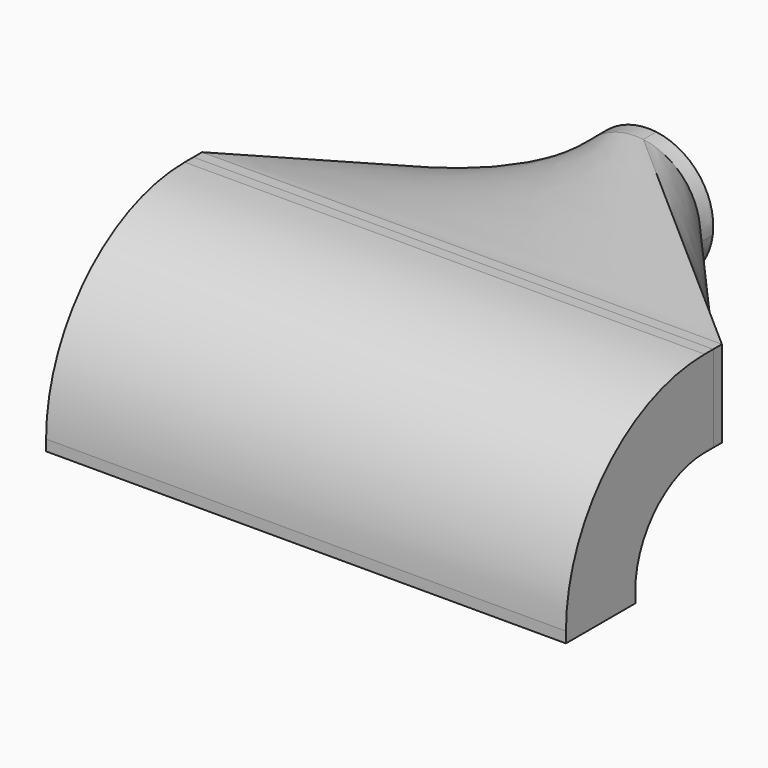
from build123d import *

# Parameters (mm, degrees)
F0_W      = 1828.8
F0_H      = 304.8
F1_DEPTH  = 38.1
F2_W      = 1828.8
F2_H      = 304.8
F3_ANGLE  = 90
F4_DEPTH  = 38.1
F5_W      = 1828.8
F5_H      = 304.8
F6_DEPTH  = 38.1
F6_FACE_W = 1828.8
F6_FACE_H = 304.8
F10_DEPTH = 57.15


# Not quite as in the source:
# - the arcs of a loft's sections are written as splines that run evenly, so that the points pair up as in the source's solid


with BuildPart() as f1:
    # F0 (on Top) → F1 (new body)
    with BuildSketch(Plane.XY):
        Rectangle(F0_W, F0_H)
    extrude(amount=F1_DEPTH)

    # F2 (on face) → F3 (revolve)
    with BuildSketch(Plane.XY.offset(38.1)):
        Rectangle(F2_W, F2_H)
    revolve(axis=Axis((-103.2055318356, 457.2, 38.1), (-1, 0, 0)), revolution_arc=F3_ANGLE)

    # F4 (add): a face of the model
    f4_faces = [f1.faces().sort_by_distance(p)[0] for p in [
        (0, 457.2, 495.3),
    ]]
    extrude(f4_faces, amount=F4_DEPTH)


with BuildPart() as f6:
    # F5 (on face) → F6 (new body)
    with BuildSketch(Plane(origin=(0, 495.3, 0), x_dir=(-1, 0, 0), z_dir=(0, 1, 0))):
        with Locations((0, 495.3)):
            Rectangle(F5_W, F5_H)
    extrude(amount=F6_DEPTH)

    # F6_face (on face) → F9 section 0
    with BuildSketch(Plane(origin=(0, 533.4, 495.3), x_dir=(-1, 0, 0), z_dir=(0, 1, 0))):
        Rectangle(F6_FACE_W, F6_FACE_H)
    # F8 (on offset) → F9 section 1
    with BuildSketch(Plane(origin=(0, 1295.4, 0), x_dir=(-1, 0, 0), z_dir=(0, 1, 0))):
        with BuildLine():
            add(Edge.make_bspline(
                [(-226.8347226167, 428.8456596729), (-224.978935382, 413.9993617947), (-221.6609974791, 399.3362055901), (-212.2280018047, 370.9382369937), (-206.1131772825, 357.2041267978), (-191.3212651368, 331.1921033689), (-182.6445432725, 318.9148333344), (-163.062159544, 296.2883825456), (-152.1569818928, 285.9397612748), (-128.5366666062, 267.5684049408), (-115.8221130296, 259.5461241455), (-89.0715816549, 246.1358631874), (-75.0362653164, 240.7482146197), (-46.1835257726, 232.8143978457), (-31.366816008, 230.2684258186), (-1.5206628948, 228.1159453578), (13.5080424489, 228.5094901485), (28.3543403271, 230.3652773833)],
                knots=[0, 0, 0, 0, 0.125, 0.125, 0.25, 0.25, 0.375, 0.375, 0.5, 0.5, 0.625, 0.625, 0.75, 0.75, 0.875, 0.875, 1, 1, 1, 1], degree=3))
            add(Edge.make_bspline(
                [(28.3543403271, 230.3652773833), (43.2006382053, 232.221064618), (57.8637944099, 235.5390025209), (86.2617630063, 244.9719981953), (99.9958732022, 251.0868227175), (126.0078966311, 265.8787348632), (138.2851666656, 274.5554567275), (160.9116174544, 294.137840456), (171.2602387252, 305.0430181072), (189.6315950592, 328.6633333938), (197.6538758545, 341.3778869704), (211.0641368126, 368.1284183451), (216.4517853803, 382.1637346836), (224.3856021543, 411.0164742274), (226.9315741814, 425.833183992), (229.0840546422, 455.6793371052), (228.6905098515, 470.7080424489), (226.8347226167, 485.5543403271)],
                knots=[0, 0, 0, 0, 0.125, 0.125, 0.25, 0.25, 0.375, 0.375, 0.5, 0.5, 0.625, 0.625, 0.75, 0.75, 0.875, 0.875, 1, 1, 1, 1], degree=3))
            add(Edge.make_bspline(
                [(226.8347226167, 485.5543403271), (224.978935382, 500.4006382053), (221.6609974791, 515.0637944099), (212.2280018047, 543.4617630063), (206.1131772825, 557.1958732022), (191.3212651368, 583.2078966311), (182.6445432725, 595.4851666656), (163.062159544, 618.1116174544), (152.1569818928, 628.4602387252), (128.5366666062, 646.8315950592), (115.8221130296, 654.8538758545), (89.0715816549, 668.2641368126), (75.0362653164, 673.6517853803), (46.1835257726, 681.5856021543), (31.366816008, 684.1315741814), (1.5206628948, 686.2840546422), (-13.5080424489, 685.8905098515), (-28.3543403271, 684.0347226167)],
                knots=[0, 0, 0, 0, 0.125, 0.125, 0.25, 0.25, 0.375, 0.375, 0.5, 0.5, 0.625, 0.625, 0.75, 0.75, 0.875, 0.875, 1, 1, 1, 1], degree=3))
            add(Edge.make_bspline(
                [(-28.3543403271, 684.0347226167), (-43.2006382053, 682.178935382), (-57.8637944099, 678.8609974791), (-86.2617630063, 669.4280018047), (-99.9958732022, 663.3131772825), (-126.0078966311, 648.5212651368), (-138.2851666656, 639.8445432725), (-160.9116174544, 620.262159544), (-171.2602387252, 609.3569818928), (-189.6315950592, 585.7366666062), (-197.6538758545, 573.0221130296), (-211.0641368126, 546.2715816549), (-216.4517853803, 532.2362653164), (-224.3856021543, 503.3835257726), (-226.9315741814, 488.566816008), (-229.0840546422, 458.7206628948), (-228.6905098515, 443.6919575511), (-226.8347226167, 428.8456596729)],
                knots=[0, 0, 0, 0, 0.125, 0.125, 0.25, 0.25, 0.375, 0.375, 0.5, 0.5, 0.625, 0.625, 0.75, 0.75, 0.875, 0.875, 1, 1, 1, 1], degree=3))
        make_face()
    loft(ruled=True)

    # F10 (add): a face of the model
    f10_faces = [f6.faces().sort_by_distance(p)[0] for p in [
        (0, 1295.4, 457.2),
    ]]
    extrude(f10_faces, amount=F10_DEPTH)


solid = Compound([f1.part, f6.part])
